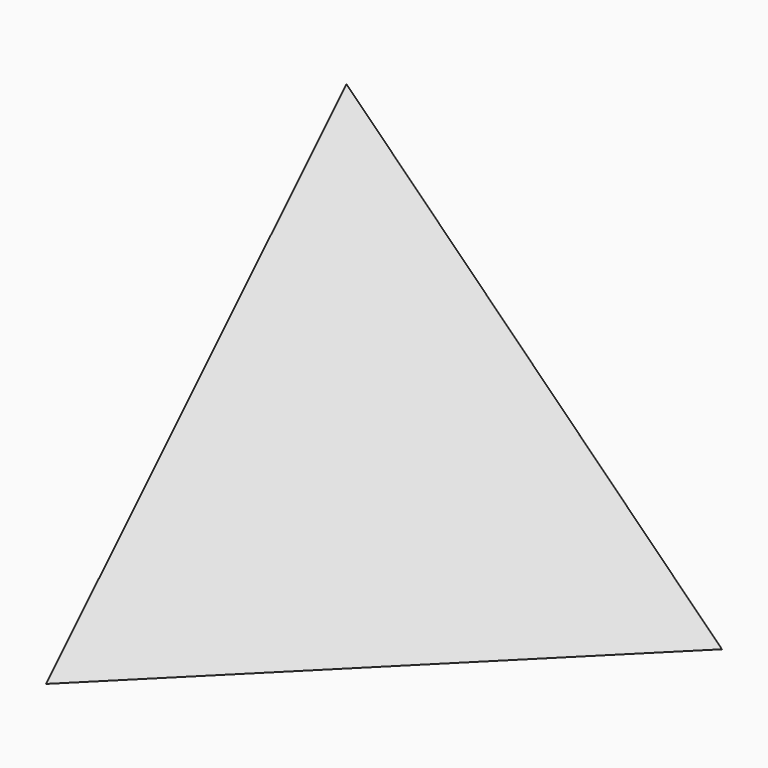
from build123d import *

# Parameters (mm, degrees)
F0_W     = 6.35
F0_H     = 6.35
F1_DEPTH = 3.175
F2_SIZE  = 6.34999


# Not quite as in the source:
# - a fillet or chamfer is up to 0.001 mm smaller than in the source, because OpenCascade refuses the exact size


with BuildPart() as f1:
    # F0 (on Right) → F1 (new body, symmetric)
    with BuildSketch(Plane.YZ):
        Rectangle(F0_W, F0_H)
    extrude(amount=F1_DEPTH, both=True)

    # F2 (size 6.35 in the source; OpenCascade refuses exactly that, so slightly less here)
    f2_edges = [f1.edges().sort_by_distance(p)[0] for p in [
        (0, -3.175, 3.175),
        (3.175, 0, 3.175),
        (3.175, -3.175, 0),
    ]]
    chamfer(f2_edges, length=F2_SIZE)


solid = f1.part
